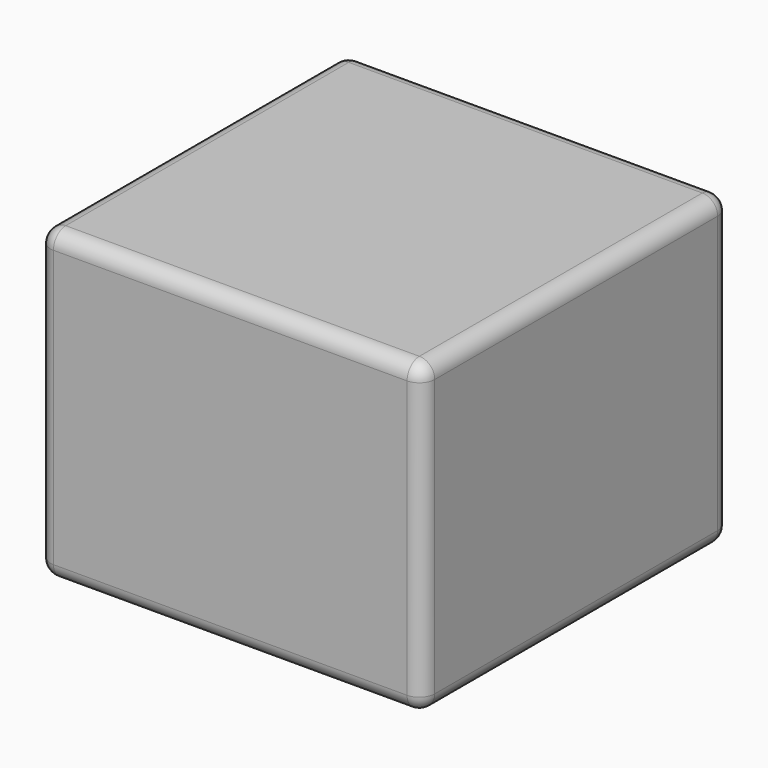
from build123d import *

# Parameters (mm, degrees)
F0_W         = 127
F0_H         = 127
F1_DEPTH     = 101.6
F2_R         = 5.08
F3_R         = 5.08
F4_T1_DEPTH  = 134.62
F4_T3_DEPTH  = 127
F4_T5_DEPTH  = 116.84
F4_S9_W      = 5.08
F4_S9_H      = 5.08
F4_T10_DEPTH = 5.08
F4_T14_ANGLE = 90
F5_T1_DEPTH  = 116.84
F5_T3_DEPTH  = 109.22
F5_S7_W      = 5.08
F5_S7_H      = 5.08
F5_T8_DEPTH  = 5.08
F5_T12_ANGLE = 90
F6_R         = 5.08


# Not quite as in the source:
# - a fillet or chamfer that OpenCascade refuses, or shapes differently, is made with other operations: its cross-section is extruded or revolved along the edge and cut away or added


with BuildPart() as f1:
    # F0 (on Top) → F1 (new body)
    with BuildSketch(Plane.XY):
        with Locations((-63.5, 63.5)):
            Rectangle(F0_W, F0_H)
    extrude(amount=F1_DEPTH)

    # F2
    f2_edges = [f1.edges().sort_by_distance(p)[0] for p in [
        (0, 63.5, 101.6),
        (0, 0, 50.8),
    ]]
    fillet(f2_edges, radius=F2_R)

    # F3
    f3_edges = [f1.edges().sort_by_distance(p)[0] for p in [
        (-127, 0, 50.8),
    ]]
    fillet(f3_edges, radius=F3_R)

    # F4: fillet of radius 5.08 on 2 edges, made by hand

    # F4_s2 → F4_t1 (cut)
    with BuildSketch(Plane.XZ.offset(-139.7)):
        with BuildLine():
            ThreePointArc((-121.92, 101.6), (-125.5121024484, 100.1121024484), (-127, 96.52))
            Line((-127, 96.52), (-127, 101.6))
            Line((-127, 101.6), (-121.92, 101.6))
        make_face()
    extrude(amount=F4_T1_DEPTH, mode=Mode.SUBTRACT)

    # F4_s4 → F4_t3 (cut)
    with BuildSketch(Plane.XY.offset(-12.7)):
        with BuildLine():
            ThreePointArc((-127, 121.92), (-125.5121024484, 125.5121024484), (-121.92, 127))
            Line((-121.92, 127), (-127, 127))
            Line((-127, 127), (-127, 121.92))
        make_face()
    extrude(amount=F4_T3_DEPTH, mode=Mode.SUBTRACT)

    # F4_s6 → F4_t5 (cut)
    with BuildSketch(Plane.YZ.offset(-121.92)):
        with BuildLine():
            ThreePointArc((0, 96.52), (1.4878975516, 100.1121024484), (5.08, 101.6))
            Line((5.08, 101.6), (0, 101.6))
            Line((0, 101.6), (0, 96.52))
        make_face()
    extrude(amount=F4_T5_DEPTH, mode=Mode.SUBTRACT)


with BuildPart() as f4_tool8:
    # F4_s9 → F4_t10 (new body)
    with BuildSketch(Plane.XZ.offset(-5.08)):
        with Locations((-2.54, 99.06)):
            Rectangle(F4_S9_W, F4_S9_H)
    extrude(amount=F4_T10_DEPTH)

    # F4_s11 → F4_t12 (revolve, cut)
    with BuildSketch(Plane(origin=(-5.08, 5.08, 96.52), x_dir=(-0.7071067812, 0, -0.7071067812), z_dir=(-0.7071067812, 0, 0.7071067812))):
        with BuildLine():
            ThreePointArc((0, -5.08), (5.08, 0), (0, 5.08))
            Line((0, 5.08), (0, -5.08))
        make_face()
    revolve(axis=Axis((-5.08, 5.08, 96.52), (0, -1, 0)), mode=Mode.SUBTRACT)


with BuildPart() as f1_1:
    add(f1.part)

    # F4_t7: cut F4_tool8
    add(f4_tool8.part, mode=Mode.SUBTRACT)

    # F4_s13 → F4_t14 (revolve, cut)
    with BuildSketch(Plane.YZ.offset(-121.92)):
        with BuildLine():
            ThreePointArc((0, 96.52), (1.4878975516, 100.1121024484), (5.08, 101.6))
            Line((5.08, 101.6), (0, 101.6))
            Line((0, 101.6), (0, 96.52))
        make_face()
    revolve(axis=Axis((-121.92, 5.08, 101.6), (0, 0, -1)), revolution_arc=F4_T14_ANGLE, mode=Mode.SUBTRACT)

    # F5: fillet of radius 5.08 on 2 edges, made by hand

    # F5_s2 → F5_t1 (cut)
    with BuildSketch(Plane.YZ.offset(-121.92)):
        with BuildLine():
            ThreePointArc((127, 96.52), (125.5121024484, 100.1121024484), (121.92, 101.6))
            Line((121.92, 101.6), (127, 101.6))
            Line((127, 101.6), (127, 96.52))
        make_face()
    extrude(amount=F5_T1_DEPTH, mode=Mode.SUBTRACT)

    # F5_s4 → F5_t3 (cut)
    with BuildSketch(Plane.XY.offset(-12.7)):
        with BuildLine():
            ThreePointArc((-5.08, 127), (-1.4878975516, 125.5121024484), (0, 121.92))
            Line((0, 121.92), (0, 127))
            Line((0, 127), (-5.08, 127))
        make_face()
    extrude(amount=F5_T3_DEPTH, mode=Mode.SUBTRACT)


with BuildPart() as f5_tool6:
    # F5_s7 → F5_t8 (new body)
    with BuildSketch(Plane.XZ.offset(-121.92)):
        with Locations((-124.46, 99.06)):
            Rectangle(F5_S7_W, F5_S7_H)
    extrude(amount=-F5_T8_DEPTH)

    # F5_s9 → F5_t10 (revolve, cut)
    with BuildSketch(Plane(origin=(-121.92, 121.92, 96.52), x_dir=(0.7071067812, 0, -0.7071067812), z_dir=(0.7071067812, 0, 0.7071067812))):
        with BuildLine():
            ThreePointArc((0, -5.08), (5.08, 0), (0, 5.08))
            Line((0, 5.08), (0, -5.08))
        make_face()
    revolve(axis=Axis((-121.92, 121.92, 96.52), (0, 1, 0)), mode=Mode.SUBTRACT)


with BuildPart() as f1_2:
    add(f1_1.part)

    # F5_t5: cut F5_tool6
    add(f5_tool6.part, mode=Mode.SUBTRACT)

    # F5_s11 → F5_t12 (revolve, cut)
    with BuildSketch(Plane.XY.offset(96.52)):
        with BuildLine():
            ThreePointArc((-5.08, 127), (-1.4878975516, 125.5121024484), (0, 121.92))
            Line((0, 121.92), (0, 127))
            Line((0, 127), (-5.08, 127))
        make_face()
    revolve(axis=Axis((-5.08, 127, 96.52), (0, -1, 0)), revolution_arc=F5_T12_ANGLE, mode=Mode.SUBTRACT)

    # F6
    f6_edges = [f1_2.edges().sort_by_distance(p)[0] for p in [
        (0, 63.5, 0),
        (-125.512102, 1.487898, 0),
        (-127, 63.5, 0),
        (-125.512102, 125.512102, 0),
        (-63.5, 127, 0),
        (-1.487898, 125.512102, 0),
        (-1.487898, 1.487898, 0),
        (-63.5, 0, 0),
    ]]
    fillet(f6_edges, radius=F6_R)


solid = f1_2.part
